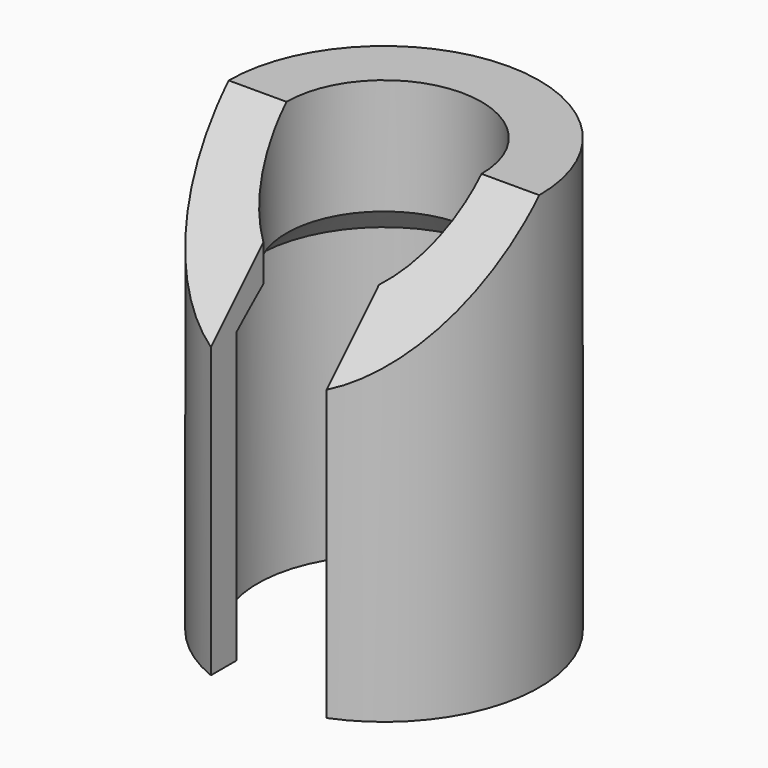
from build123d import *

# Parameters (mm, degrees)
F1_DEPTH      = 10
F3_DEPTH      = 5
F4_SIZE       = 0.99999
F6_DEPTH      = 25
F6_DEPTH_BACK = 25


# Not quite as in the source:
# - a fillet or chamfer is up to 0.001 mm smaller than in the source, because OpenCascade refuses the exact size


with BuildPart() as f1:
    # F0 (on Top) → F1 (new body)
    with BuildSketch(Plane.XY):
        with BuildLine():
            Line((2, -3.8910956041), (2, -4.9890505109))
            ThreePointArc((2, -4.9890505109), (0, 5.375), (-2, -4.9890505109))
            Line((-2, -4.9890505109), (-2, -3.8910956041))
            ThreePointArc((-2, -3.8910956041), (0, 4.375), (2, -3.8910956041))
        make_face()
    extrude(amount=F1_DEPTH)

    # F2 (on face) → F3 (join)
    with BuildSketch(Plane.XY.offset(10)):
        with BuildLine():
            Line((2, -2.7185703964), (2, -4.9890505109))
            ThreePointArc((2, -4.9890505109), (0, 5.375), (-2, -4.9890505109))
            Line((-2, -4.9890505109), (-2, -2.7185703964))
            ThreePointArc((-2, -2.7185703964), (0, 3.375), (2, -2.7185703964))
        make_face()
    extrude(amount=F3_DEPTH)

    # F4 (size 1 in the source; OpenCascade refuses exactly that, so slightly less here)
    f4_edges = [f1.edges().sort_by_distance(p)[0] for p in [
        (0, 3.375, 10),
    ]]
    chamfer(f4_edges, length=F4_SIZE)

    # F5 (on Right) → F6 (cut, two sides)
    with BuildSketch(Plane.YZ) as f6_sk:
        Polygon((0, 15), (-4.9890505109, 15), (-4.9890505109, 10), align=None)
    extrude(amount=-F6_DEPTH, mode=Mode.SUBTRACT)
    extrude(f6_sk.sketch, amount=F6_DEPTH_BACK, mode=Mode.SUBTRACT)


solid = f1.part
